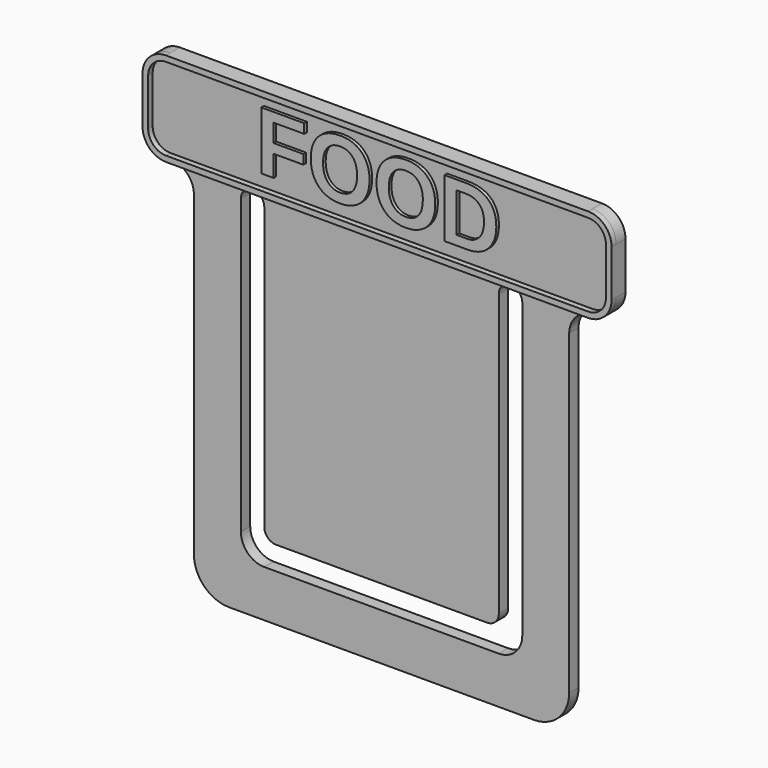
from build123d import *

# Parameters (mm, degrees)
F0_W          = 25.4
F0_H          = 25.4
F1_DEPTH      = 0.79375
F2_R          = 2.38125
F3_W          = 19.05
F3_H          = 22.225
F4_DEPTH      = 4.9276
F6_DEPTH      = 0.79375
F7_R          = 1.58749
F8_R          = 1.5875
F9_W          = 15.875
F9_H          = 20.6375
F10_DEPTH     = 0.79375
F11_R         = 0.79374
F12_R         = 0.79375
F14_DEPTH     = 0.381
F16_DEPTH     = 0.381
F17_TEXT_SIZE = 5.7207213508
F18_DEPTH     = 1.016


# Not quite as in the source:
# - a fillet or chamfer is up to 0.001 mm smaller than in the source, because OpenCascade refuses the exact size
# - ends of sketch curves that miss each other by under 0.0002 mm in the source are joined
# - Text() gives the source's letters only with a copy of the font that has no kerning and outlines rounded to 1/6400 em; it was checked with that copy


with BuildPart() as f1:
    # F0 (on Front) → F1 (new body)
    with BuildSketch(Plane.XZ):
        Rectangle(F0_W, F0_H)
    extrude(amount=F1_DEPTH)

    # F2
    f2_edges = [f1.edges().sort_by_distance(p)[0] for p in [
        (12.7, -0.396875, -12.7),
        (-12.7, -0.396875, -12.7),
    ]]
    fillet(f2_edges, radius=F2_R)

    # F3 (on face) → F4 (cut)
    with BuildSketch(Plane.XZ.offset(0.79375)):
        with Locations((0, 1.5875)):
            Rectangle(F3_W, F3_H)
    extrude(amount=-F4_DEPTH, mode=Mode.SUBTRACT)

    # F5 (on face) → F6 (join)
    with BuildSketch(Plane.XZ.offset(0.79375)):
        Polygon((-15.875, 19.05), (-15.875, 12.7), (-12.7, 12.7), (-9.525, 12.7), (9.525, 12.7), (12.7, 12.7), (15.875, 12.7), (15.875, 19.05), align=None)
    extrude(amount=-F6_DEPTH)

    # F7 (radius 1.5875 in the source; OpenCascade refuses exactly that, so slightly less here)
    f7_edges = [f1.edges().sort_by_distance(p)[0] for p in [
        (-15.875, -0.396875, 19.05),
        (15.875, -0.396875, 19.05),
        (15.875, -0.396875, 12.7),
        (12.7, -0.396875, 12.7),
        (-15.875, -0.396875, 12.7),
        (-12.7, -0.396875, 12.7),
    ]]
    fillet(f7_edges, radius=F7_R)

    # F8
    f8_edges = [f1.edges().sort_by_distance(p)[0] for p in [
        (-9.525, -0.396875, -9.525),
        (9.525, -0.396875, -9.525),
    ]]
    fillet(f8_edges, radius=F8_R)

    # F9 (on face) → F10 (join)
    with BuildSketch(Plane.XZ.offset(0.79375)):
        with BuildLine():
            ThreePointArc((-14.28751, 19.05), (-15.4100349441, 18.5850349441), (-15.875, 17.46251))
            Line((-15.875, 17.46251), (-15.875, 14.28749))
            ThreePointArc((-15.875, 14.28749), (-15.4100349441, 13.1649650559), (-14.28751, 12.7))
            ThreePointArc((-14.28751, 12.7), (-13.1649650559, 12.2350349441), (-12.7, 11.11251))
            Line((-12.7, 11.11251), (-12.7, -10.31875))
            ThreePointArc((-12.7, -10.31875), (-12.0025480227, -12.0025480227), (-10.31875, -12.7))
            Line((-10.31875, -12.7), (10.31875, -12.7))
            ThreePointArc((10.31875, -12.7), (12.0025480227, -12.0025480227), (12.7, -10.31875))
            Line((12.7, -10.31875), (12.7, 11.11251))
            ThreePointArc((12.7, 11.11251), (13.1649650559, 12.2350349441), (14.28749, 12.7))
            ThreePointArc((14.28749, 12.7), (15.4100349441, 13.1649650559), (15.875, 14.28749))
            Line((15.875, 14.28749), (15.875, 17.46251))
            ThreePointArc((15.875, 17.46251), (15.4100349441, 18.5850349441), (14.28751, 19.05))
            Line((14.28751, 19.05), (-14.28751, 19.05))
        make_face()
        with BuildLine():
            Line((-9.525, 12.7), (-7.9375, 12.7))
            Line((-7.9375, 12.7), (7.9375, 12.7))
            Line((7.9375, 12.7), (9.525, 12.7))
            Line((9.525, 12.7), (9.525, -7.9375))
            ThreePointArc((9.525, -7.9375), (9.0600320151, -9.0600320151), (7.9375, -9.525))
            Line((7.9375, -9.525), (-7.9375, -9.525))
            ThreePointArc((-7.9375, -9.525), (-9.0600320151, -9.0600320151), (-9.525, -7.9375))
            Line((-9.525, -7.9375), (-9.525, 12.7))
        make_face(mode=Mode.SUBTRACT)
        with Locations((0, 2.38125)):
            Rectangle(F9_W, F9_H)
    extrude(amount=-F10_DEPTH)

    # F11 (radius 0.79375 in the source; OpenCascade refuses exactly that, so slightly less here)
    f11_edges = [f1.edges().sort_by_distance(p)[0] for p in [
        (-7.9375, -0.396875, 12.7),
        (-9.525, -0.396875, 12.7),
        (7.9375, -0.396875, 12.7),
        (9.525, -0.396875, 12.7),
    ]]
    fillet(f11_edges, radius=F11_R)

    # F12
    f12_edges = [f1.edges().sort_by_distance(p)[0] for p in [
        (-7.9375, -0.396875, -7.9375),
        (7.9375, -0.396875, -7.9375),
    ]]
    fillet(f12_edges, radius=F12_R)

    # F13 (on face) → F14 (join)
    with BuildSketch(Plane.XZ.offset(0.79375)):
        with BuildLine():
            Line((14.2875, 19.05), (-14.2875, 19.05))
            ThreePointArc((-14.2875, 19.05), (-15.4100320151, 18.5850320151), (-15.875, 17.4625))
            Line((-15.875, 17.4625), (-15.875, 14.2875))
            ThreePointArc((-15.875, 14.2875), (-15.4100320151, 13.1649679849), (-14.2875, 12.7))
            Line((-14.2875, 12.7), (-8.73125, 12.7))
            Line((-8.73125, 12.7), (8.73125, 12.7))
            Line((8.73125, 12.7), (14.2875, 12.7))
            ThreePointArc((14.2875, 12.7), (15.4100320151, 13.1649679849), (15.875, 14.2875))
            Line((15.875, 14.2875), (15.875, 17.4625))
            ThreePointArc((15.875, 17.4625), (15.4100320151, 18.5850320151), (14.2875, 19.05))
        make_face()
    extrude(amount=F14_DEPTH)

    # F15 (on face) → F16 (cut, through all)
    with BuildSketch(Plane.XZ.offset(1.17475)):
        with BuildLine():
            Line((14.2875, 18.669), (-14.2875, 18.669))
            ThreePointArc((-14.2875, 18.669), (-15.1406243315, 18.3156243315), (-15.494, 17.4625))
            Line((-15.494, 17.4625), (-15.494, 14.2875))
            ThreePointArc((-15.494, 14.2875), (-15.1406243315, 13.4343756685), (-14.2875, 13.081))
            Line((-14.2875, 13.081), (14.2875, 13.081))
            ThreePointArc((14.2875, 13.081), (15.1406243315, 13.4343756685), (15.494, 14.2875))
            Line((15.494, 14.2875), (15.494, 17.4625))
            ThreePointArc((15.494, 17.4625), (15.1406243315, 18.3156243315), (14.2875, 18.669))
        make_face()
    extrude(amount=-F16_DEPTH, mode=Mode.SUBTRACT)

    # F17 (on Front) → F18 (join)
    with BuildSketch(Plane.XZ):
        with Locations((-8.3406329569, 14.010136947)):
            Text('FOOD', F17_TEXT_SIZE, font='Arimo', font_style=FontStyle.BOLD, text_align=(TextAlign.LEFT, TextAlign.BOTTOM))
    extrude(amount=F18_DEPTH)


solid = f1.part
